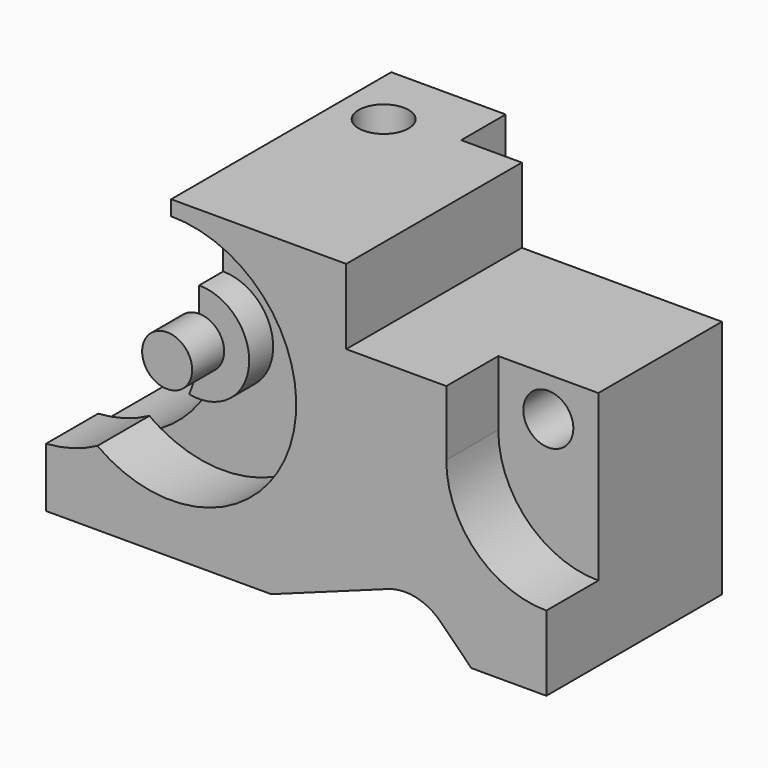
from build123d import *

# Parameters (mm, degrees)
F1_DEPTH  = 42
F3_DEPTH  = 6
F4_R      = 5
F5_DEPTH  = 8
F7_DEPTH  = 13
F8_R      = 5
F9_DEPTH  = 100
F10_W     = 54.9314450473
F10_H     = 11.126392521
F11_DEPTH = 100
F12_R     = 5
F13_DEPTH = 100
F14_W     = 30.3172562271
F14_H     = 20.0113151222
F15_DEPTH = 30
F16_W     = 11.4489658736
F16_H     = 47.9527432472
F17_DEPTH = 30
F18_W     = 14.1378343105
F18_H     = 19.7980464436
F19_DEPTH = 24


with BuildPart() as f1:
    # F0 (on Front) → F1 (new body)
    with BuildSketch(Plane.XZ):
        with BuildLine():
            Line((-25, -25), (-25, -35))
            Line((-25, -35), (20, -35))
            Line((20, -35), (43.3396509331, -26.5050617822))
            ThreePointArc((43.3396509331, -26.5050617822), (48.9242485057, -26.1390279189), (53.8309201782, -28.8309201782))
            Line((53.8309201782, -28.8309201782), (60, -35))
            Line((60, -35), (75, -35))
            Line((75, -35), (75, 13))
            Line((75, 13), (35, 13))
            Line((35, 13), (35, 28))
            Line((35, 28), (0, 28))
            Line((0, 28), (0, 0))
            ThreePointArc((0, 0), (-7.3223304703, -17.6776695297), (-25, -25))
        make_face()
    extrude(amount=F1_DEPTH)

    # F2 (on face) → F3 (join)
    with BuildSketch(Plane.XZ.offset(42)):
        with BuildLine():
            ThreePointArc((0, 0), (-0.5051025722, -5), (-2, -9.7979589711))
            ThreePointArc((-2, -9.7979589711), (9.9493615301, -1.0050896201), (0, 10))
            Line((0, 10), (0, 0))
        make_face()
    extrude(amount=F3_DEPTH)

    # F4 (on face) → F5 (join)
    with BuildSketch(Plane.XZ.offset(48)):
        Circle(F4_R)
    extrude(amount=F5_DEPTH)

    # F6 (on face) → F7 (join)
    with BuildSketch(Plane.XZ.offset(42)):
        with BuildLine():
            ThreePointArc((0, 25), (23.7688536403, -7.7486512779), (-14.7341246507, -20.1966722699))
            ThreePointArc((-14.7341246507, -20.1966722699), (-19.7077962092, -22.2252520213), (-25, -23.1445580721))
            Line((-25, -23.1445580721), (-25, -35))
            Line((-25, -35), (20, -35))
            Line((20, -35), (43.3396509331, -26.5050617822))
            ThreePointArc((43.3396509331, -26.5050617822), (48.9242485057, -26.1390279189), (53.8309201782, -28.8309201782))
            Line((53.8309201782, -28.8309201782), (60, -35))
            Line((60, -35), (75, -35))
            Line((75, -35), (75, -20))
            ThreePointArc((75, -20), (60.8578643763, -14.1421356237), (55, 0))
            Line((55, 0), (55, 13))
            Line((55, 13), (35, 13))
            Line((35, 13), (35, 28))
            Line((35, 28), (0, 28))
            Line((0, 28), (0, 25))
        make_face()
    extrude(amount=F7_DEPTH)

    # F8 (on face) → F9 (cut)
    with BuildSketch(Plane.XZ.offset(42)):
        with Locations((65, 5.1525061529)):
            Circle(F8_R)
    extrude(amount=-F9_DEPTH, mode=Mode.SUBTRACT)

    # F10 (on face) → F11 (cut)
    with BuildSketch(Plane.XY.offset(28)):
        with Locations((50.3426203504, -5.5631962605)):
            Rectangle(F10_W, F10_H)
    extrude(amount=-F11_DEPTH, mode=Mode.SUBTRACT)

    # F12 (on face) → F13 (cut)
    with BuildSketch(Plane.XY.offset(28)):
        with Locations((9, -13.1446226788)):
            Circle(F12_R)
    extrude(amount=-F13_DEPTH, mode=Mode.SUBTRACT)

    # F14 (on face) → F15 (cut)
    with BuildSketch(Plane(origin=(0, -11.126392521, 0), x_dir=(-1, 0, 0), z_dir=(0, 1, 0))):
        with Locations((-42.6998464391, -10.0056575611)):
            Rectangle(F14_W, F14_H)
    extrude(amount=-F15_DEPTH, mode=Mode.SUBTRACT)

    # F16 (on face) → F17 (cut)
    with BuildSketch(Plane(origin=(0, 0, 0), x_dir=(-1, 0, 0), z_dir=(0, 1, 0))):
        with Locations((-11.9378056843, -5.1767108962)):
            Rectangle(F16_W, F16_H)
    extrude(amount=-F17_DEPTH, mode=Mode.SUBTRACT)

    # F18 (on face) → F19 (cut)
    with BuildSketch(Plane(origin=(0, -11.126392521, 0), x_dir=(-1, 0, 0), z_dir=(0, 1, 0))):
        with Locations((-64.9273917079, -16.0573225003)):
            Rectangle(F18_W, F18_H)
    extrude(amount=-F19_DEPTH, mode=Mode.SUBTRACT)


solid = f1.part
